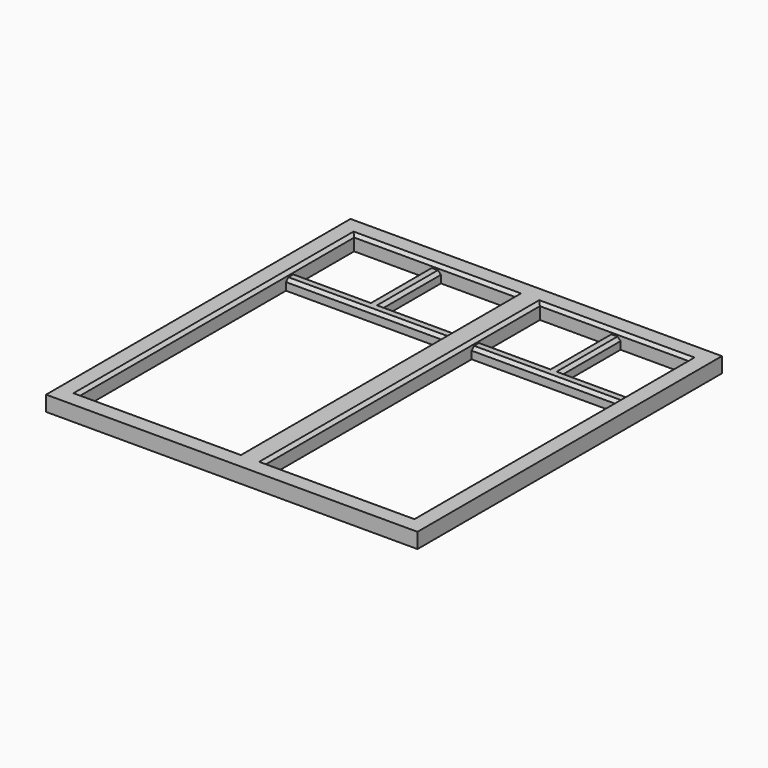
from build123d import *

# Parameters (mm, degrees)
F0_W      = 1220
F0_H      = 1250
F1_DEPTH  = 50
F2_DEPTH  = 35
F3_SIZE   = 10
F3_2_SIZE = 10
F3_3_SIZE = 10


with BuildPart() as f1:
    # F0 (on Top) → F1 (new body)
    with BuildSketch(Plane.XY):
        with Locations((200.3141621128, 70.2047318473)):
            Rectangle(F0_W, F0_H)
        Polygon((-349.6858378872, -494.7952681527), (-349.6858378872, 355.2047318473), (-349.6858378872, 395.2047318473), (-349.6858378872, 635.2047318473), (-104.6858378872, 635.2047318473), (-64.6858378872, 635.2047318473), (180.3141621128, 635.2047318473), (180.3141621128, 395.2047318473), (180.3141621128, 355.2047318473), (180.3141621128, -494.7952681527), align=None, mode=Mode.SUBTRACT)
        Polygon((260.3141621128, -494.7952681527), (260.3141621128, 355.2047318473), (260.3141621128, 395.2047318473), (260.3141621128, 635.2047318473), (485.3141621128, 635.2047318473), (525.3141621128, 635.2047318473), (750.3141621128, 635.2047318473), (750.3141621128, 395.2047318473), (750.3141621128, 355.2047318473), (750.3141621128, -494.7952681527), align=None, mode=Mode.SUBTRACT)
    extrude(amount=F1_DEPTH)

    # F3
    f3_edges = [f1.edges().sort_by_distance(p)[0] for p in [
        (-349.685838, 70.204732, 50),
        (-84.685838, 635.204732, 50),
        (180.314162, 70.204732, 50),
        (260.314162, 70.204732, 50),
        (505.314162, 635.204732, 50),
        (750.314162, 70.204732, 50),
        (505.314162, -494.795268, 50),
        (-84.685838, -494.795268, 50),
    ]]
    chamfer(f3_edges, length=F3_SIZE)


with BuildPart() as f2:
    # F0 (on Top) → F2 (new body)
    with BuildSketch(Plane.XY):
        Polygon((-349.6858378872, 395.2047318473), (-349.6858378872, 355.2047318473), (180.3141621128, 355.2047318473), (180.3141621128, 395.2047318473), (-64.6858378872, 395.2047318473), (-64.6858378872, 635.2047318473), (-104.6858378872, 635.2047318473), (-104.6858378872, 395.2047318473), align=None)
    extrude(amount=F2_DEPTH)

    # F3#2
    f3_2_edges = [f2.edges().sort_by_distance(p)[0] for p in [
        (-84.685838, 355.204732, 35),
        (57.814162, 395.204732, 35),
        (-64.685838, 515.204732, 35),
        (-104.685838, 515.204732, 35),
        (-227.185838, 395.204732, 35),
    ]]
    chamfer(f3_2_edges, length=F3_2_SIZE)


with BuildPart() as f2b:
    # F0 (on Top) → F2, piece 2 (new body)
    with BuildSketch(Plane.XY):
        Polygon((260.3141621128, 395.2047318473), (260.3141621128, 355.2047318473), (750.3141621128, 355.2047318473), (750.3141621128, 395.2047318473), (525.3141621128, 395.2047318473), (525.3141621128, 635.2047318473), (485.3141621128, 635.2047318473), (485.3141621128, 395.2047318473), align=None)
    extrude(amount=F2_DEPTH)

    # F3#3
    f3_3_edges = [f2b.edges().sort_by_distance(p)[0] for p in [
        (505.314162, 355.204732, 35),
        (372.814162, 395.204732, 35),
        (525.314162, 515.204732, 35),
        (637.814162, 395.204732, 35),
        (485.314162, 515.204732, 35),
    ]]
    chamfer(f3_3_edges, length=F3_3_SIZE)


solid = Compound([f1.part, f2.part, f2b.part])
